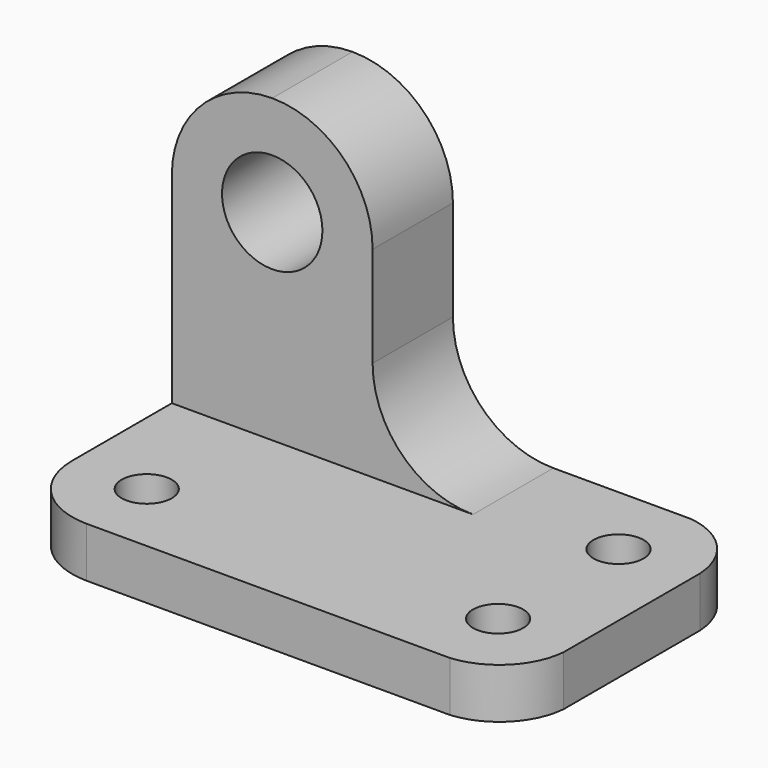
from build123d import *

# Parameters (mm, degrees)
F0_W      = 63.5
F0_H      = 44.45
F1_DEPTH  = 38.1
F2_W      = 25.4
F2_H      = 38.1
F3_DEPTH  = 38.101
F5_W      = 25.4
F5_H      = 38.1
F6_DEPTH  = 38.101
F4_W      = 12.7
F4_H      = 25.4
F7_DEPTH  = 38.101
F8_R      = 6.35
F9_DEPTH  = 12.701
F10_R     = 3.175
F11_DEPTH = 6.351


# Not quite as in the source:
# - a feature names something its author has since deleted; it is built from what else it names


with BuildPart() as f1:
    # F0 (on Front) → F1 (new body)
    with BuildSketch(Plane.XZ):
        with Locations((31.75, 22.225)):
            Rectangle(F0_W, F0_H)
    extrude(amount=F1_DEPTH)

    # F2 (on face) → F3 (cut, through all)
    with BuildSketch(Plane.XZ.offset(38.1)):
        with Locations((50.8, 25.4)):
            Rectangle(F2_W, F2_H)
    extrude(amount=-F3_DEPTH, mode=Mode.SUBTRACT)

    # F5 (on face) → F6 (cut, through all)
    with BuildSketch(Plane.YZ.offset(38.1)):
        with Locations((-25.4, 25.4)):
            Rectangle(F5_W, F5_H)
    extrude(amount=-F6_DEPTH, mode=Mode.SUBTRACT)

    # F4 (on face) → F7 (cut, through all)
    with BuildSketch(Plane.XZ.offset(38.1)):
        with Locations((31.75, 31.75)):
            Rectangle(F4_W, F4_H)
        with BuildLine():
            Line((38.1, 19.05), (25.4, 19.05))
            ThreePointArc((25.4, 19.05), (29.1197438789, 10.0697438789), (38.1, 6.35))
            Line((38.1, 6.35), (38.1, 19.05))
        make_face()
    extrude(amount=-F7_DEPTH, mode=Mode.SUBTRACT)

    # F8 (on face) → F9 (cut, through all)
    with BuildSketch(Plane.XZ.offset(12.7)):
        with Locations((12.7, 31.75)):
            Circle(F8_R)
        with BuildLine():
            ThreePointArc((12.6999999213, 44.45), (21.6802560932, 40.7302561489), (25.4, 31.75))
            Line((25.4, 31.75), (25.4, 44.45))
            Line((25.4, 44.45), (12.6999999213, 44.45))
        make_face()
        with BuildLine():
            ThreePointArc((0, 31.75), (3.7197438511, 40.7302560932), (12.6999999213, 44.45))
            Line((12.6999999213, 44.45), (0, 44.45))
            Line((0, 44.45), (0, 31.75))
        make_face()
    extrude(amount=-F9_DEPTH, mode=Mode.SUBTRACT)

    # F10 (on face) → F11 (cut, through all)
    with BuildSketch(Plane.XY.offset(6.35)):
        with BuildLine():
            Line((63.5, 0), (55.5319362459, 0))
            ThreePointArc((55.5319362459, 0), (61.0732443905, -2.8419244619), (63.5, -8.5772089198))
            Line((63.5, -8.5772089198), (63.5, 0))
        make_face()
        with BuildLine():
            ThreePointArc((63.5, -30.1359133542), (60.963360935, -35.563360935), (55.5359133542, -38.1))
            Line((55.5359133542, -38.1), (63.5, -38.1))
            Line((63.5, -38.1), (63.5, -30.1359133542))
        make_face()
        with BuildLine():
            ThreePointArc((9.525, -38.1), (2.8223237752, -35.2776762248), (0, -28.575))
            Line((0, -28.575), (0, -38.1))
            Line((0, -38.1), (9.525, -38.1))
        make_face()
        with Locations((9.525, -28.575)):
            Circle(F10_R)
        with Locations((53.975, -28.575)):
            Circle(F10_R)
        with Locations((53.975, -9.525)):
            Circle(F10_R)
    extrude(amount=-F11_DEPTH, mode=Mode.SUBTRACT)


solid = f1.part
